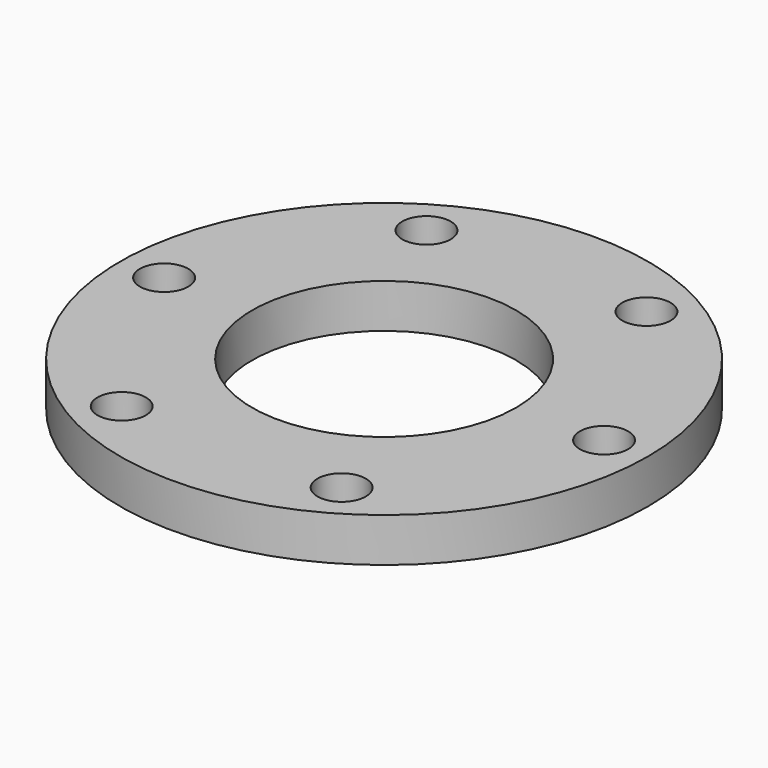
from build123d import *

# Parameters (mm, degrees)
F0_R            = 60
F0_R_2          = 30
F1_DEPTH        = 10
F3_D            = 11
F3_COPIES_COUNT = 6


# Not quite as in the source:
# - a pattern or mirror of a feature is missing from the dataset's text; its kind, count and spacing are read off the source's solid


with BuildPart() as f1:
    # F0 (on Top) → F1 (new body)
    with BuildSketch(Plane.XY):
        Circle(F0_R)
        Circle(F0_R_2, mode=Mode.SUBTRACT)
    extrude(amount=F1_DEPTH)

    # F3 (through all)
    with Locations(Plane.XY.offset(10)):
        with Locations((-50, 0)):
            f3 = Hole(F3_D / 2)

    # F3_copies: F3 ×6 about axis
    f3_copies_axis = Axis((0, 0, 0), (0, 0, 1))
    for i in range(1, F3_COPIES_COUNT):
        add(f3.rotate(f3_copies_axis, i * 360 / F3_COPIES_COUNT), mode=Mode.SUBTRACT)


solid = f1.part
